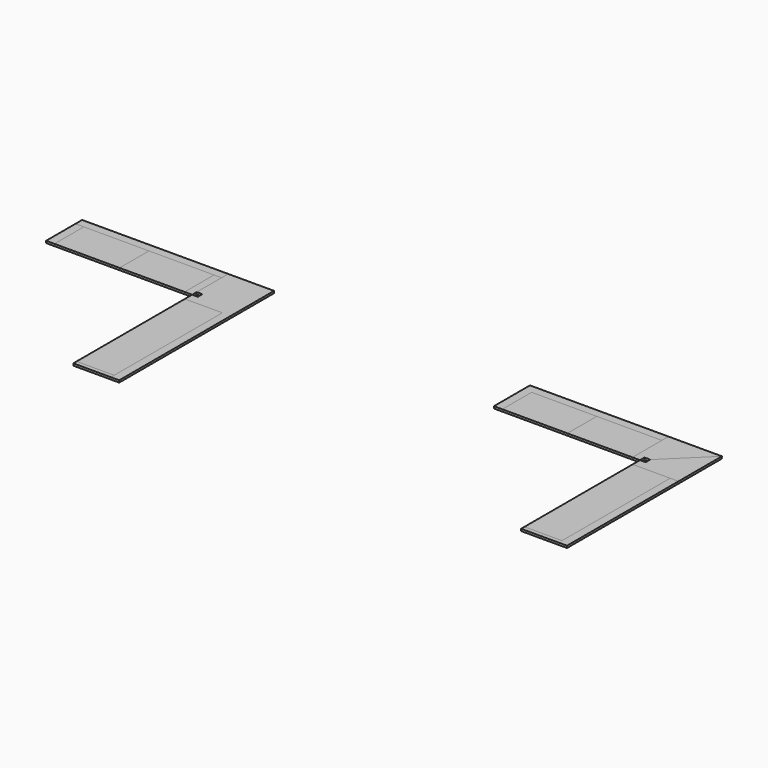
from build123d import *

# Parameters (mm, degrees)
F0_W     = 100
F0_H     = 440
F1_DEPTH = 25
F0_W_2   = 780
F0_W_3   = 450
F0_H_2   = 50
F2_DEPTH = 25
F0_H_3   = 1620
F3_DEPTH = 25
F4_DEPTH = 25
F6_W     = 10
F6_H     = 7
F7_REACH = 7112.0815171795


with BuildPart() as f1:
    # F0 (on Top) → F1 (new body)
    with BuildSketch(Plane.XY):
        with Locations((-1700, 220)):
            Rectangle(F0_W, F0_H)
    extrude(amount=F1_DEPTH)


with BuildPart() as f1b:
    # F0 (on Top) → F1, piece 2 (new body)
    with BuildSketch(Plane.XY):
        with Locations((-480, 220)):
            Rectangle(F0_W_2, F0_H)
    extrude(amount=F1_DEPTH)


with BuildPart() as f1c:
    # F0 (on Top) → F1, piece 3 (new body)
    with BuildSketch(Plane.XY):
        with Locations((225, -1755)):
            Rectangle(F0_W_3, F0_H_2)
    extrude(amount=F1_DEPTH)


with BuildPart() as f1d:
    # F0 (on Top) → F1, piece 4 (new body)
    with BuildSketch(Plane.XY):
        Polygon((4495.2596473694, 440.0000286102), (5275.2596473694, 440.0000286102), (5275.2596473694, 540.0000286102), (3615.2596473694, 540.0000286102), (3615.2596473694, 2.86102e-05), (3715.2596473694, 2.86102e-05), (3715.2596473694, 440.0000286102), align=None)
    extrude(amount=F1_DEPTH)


with BuildPart() as f1e:
    # F0 (on Top) → F1, piece 5 (new body)
    with BuildSketch(Plane.XY):
        Polygon((5433.2596473694, 2.86102e-05), (5365.2596473694, 2.86102e-05), (5365.2596473694, -109.9999713898), (5815.2596473694, -109.9999713898), (5915.2596473694, -109.9999713898), (5915.2596473694, 540.0000286102), (5433.2596473694, 68.0000286102), align=None)
    extrude(amount=F1_DEPTH)


with BuildPart() as f2:
    # F0 (on Top) → F2 (new body)
    with BuildSketch(Plane.XY):
        Polygon((550, -110), (450, -110), (450, -1730), (450, -1780), (550, -1780), align=None)
        Polygon((68, 0), (0, 0), (0, -110), (450, -110), (550, -110), (550, 540), (0, 540), (0, 440), (0, 68), (68, 68), align=None)
    extrude(amount=F2_DEPTH)


with BuildPart() as f2b:
    # F0 (on Top) → F2, piece 2 (new body)
    with BuildSketch(Plane.XY):
        with Locations((-1260, 220)):
            Rectangle(F0_W_2, F0_H)
    extrude(amount=F2_DEPTH)


with BuildPart() as f2c:
    # F0 (on Top) → F2, piece 3 (new body)
    with BuildSketch(Plane.XY):
        with Locations((4105.2596473694, 220.0000286102)):
            Rectangle(F0_W_2, F0_H)
    extrude(amount=F2_DEPTH)


with BuildPart() as f2d:
    # F0 (on Top) → F2, piece 4 (new body)
    with BuildSketch(Plane.XY):
        Polygon((5275.2596473694, 2.86102e-05), (5365.2596473694, 2.86102e-05), (5365.2596473694, 68.0000286102), (5433.2596473694, 68.0000286102), (5915.2596473694, 540.0000286102), (5275.2596473694, 540.0000286102), (5275.2596473694, 440.0000286102), align=None)
    extrude(amount=F2_DEPTH)


with BuildPart() as f2e:
    # F0 (on Top) → F2, piece 5 (new body)
    with BuildSketch(Plane.XY):
        with Locations((5590.2596473694, -919.9999713898)):
            Rectangle(F0_W_3, F0_H_3)
    extrude(amount=F2_DEPTH)


with BuildPart() as f3:
    # F0 (on Top) → F3 (new body)
    with BuildSketch(Plane.XY):
        with Locations((225, -920)):
            Rectangle(F0_W_3, F0_H_3)
    extrude(amount=F3_DEPTH)


with BuildPart() as f3b:
    # F0 (on Top) → F3, piece 2 (new body)
    with BuildSketch(Plane.XY):
        Polygon((-90, 440), (0, 440), (0, 540), (-1750, 540), (-1750, 440), (-1650, 440), (-870, 440), align=None)
    extrude(amount=F3_DEPTH)


with BuildPart() as f3c:
    # F0 (on Top) → F3, piece 3 (new body)
    with BuildSketch(Plane.XY):
        Polygon((5915.2596473694, -109.9999713898), (5815.2596473694, -109.9999713898), (5815.2596473694, -1729.9999713898), (5365.2596473694, -1729.9999713898), (5365.2596473694, -1779.9999713898), (5915.2596473694, -1779.9999713898), align=None)
    extrude(amount=F3_DEPTH)


with BuildPart() as f3d:
    # F0 (on Top) → F3, piece 4 (new body)
    with BuildSketch(Plane.XY):
        with Locations((4885.2596473694, 220.0000286102)):
            Rectangle(F0_W_2, F0_H)
    extrude(amount=F3_DEPTH)


with BuildPart() as f4:
    # F0 (on Top) → F4 (new body)
    with BuildSketch(Plane.XY):
        Polygon((-90, 0), (0, 0), (0, 68), (0, 440), (-90, 440), align=None)
    extrude(amount=F4_DEPTH)


with BuildPart() as f7:
    f7_end = Plane(origin=(5399.2596473694, 68.0000286102, 12.5), x_dir=(0, 0, -1), z_dir=(0, -1, 0))
    # F6 (on face) → F7 (new body, up to a plane its end follows)
    with BuildSketch(Plane(origin=(3289.5685174165, 3221.3202079265, 0), x_dir=(-0.6996563237, 0.7144795509, 0), z_dir=(0.7144795509, 0.6996563237, 0))):
        with Locations((-3747.8298407898, 12.5)):
            Rectangle(F6_W, F6_H)
        with Locations((-3757.8298407898, 12.5)):
            Rectangle(F6_W, F6_H)
    f7_long = extrude(amount=-F7_REACH, mode=Mode.PRIVATE)
    add(split(f7_long, bisect_by=f7_end, keep=Keep.BOTTOM, mode=Mode.PRIVATE))


with BuildPart() as f2d_1:
    add(f2d.part)

    # F8: cut F7
    add(f7.part, mode=Mode.SUBTRACT)


with BuildPart() as f1e_1:
    add(f1e.part)

    # F8: cut F7
    add(f7.part, mode=Mode.SUBTRACT)


solid = Compound([f1.part, f1b.part, f1c.part, f1d.part, f2.part, f2b.part, f2c.part, f2e.part, f3.part, f3b.part, f3c.part, f3d.part, f4.part, f2d_1.part, f1e_1.part])
